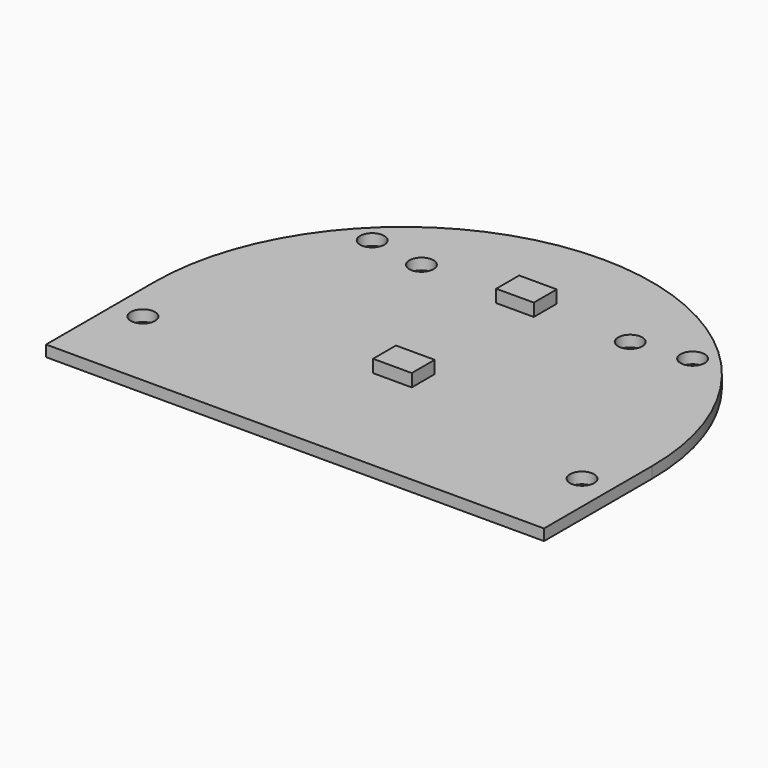
from build123d import *

# Parameters (mm, degrees)
F0_W     = 66.9
F0_H     = 51.6
F1_DEPTH = 1.5
F2_R     = 33.44999
F3_R     = 1.625
F4_DEPTH = 1.5
F5_W     = 5.2
F5_H     = 3.85
F5_W_2   = 5.05
F6_DEPTH = 1.7


# Not quite as in the source:
# - a fillet or chamfer is up to 0.001 mm smaller than in the source, because OpenCascade refuses the exact size


with BuildPart() as f1:
    # F0 (on Top) → F1 (new body)
    with BuildSketch(Plane.XY):
        Rectangle(F0_W, F0_H)
    extrude(amount=F1_DEPTH)

    # F2 (radius 33.45 in the source; OpenCascade refuses exactly that, so slightly less here)
    f2_edges = [f1.edges().sort_by_distance(p)[0] for p in [
        (-33.45, 25.8, 0.75),
        (33.45, 25.8, 0.75),
    ]]
    fillet(f2_edges, radius=F2_R)

    # F3 (on Top) → F4 (cut)
    with BuildSketch(Plane.XY):
        with Locations((-21.525, 14.0641658831)):
            Circle(F3_R)
        with Locations((-14.025, 12.9547324661)):
            Circle(F3_R)
        with Locations((21.525, 14.0641658831)):
            Circle(F3_R)
        with Locations((14.025, 12.9547324661)):
            Circle(F3_R)
        with Locations((-29.5, -14.475)):
            Circle(F3_R)
        with Locations((29.5, -14.475)):
            Circle(F3_R)
    extrude(amount=F4_DEPTH, mode=Mode.SUBTRACT)

    # F5 (on face) → F6 (join)
    with BuildSketch(Plane.XY.offset(1.5)):
        with Locations((0, -7.525)):
            Rectangle(F5_W, F5_H)
        with Locations((0.075, 12.975)):
            Rectangle(F5_W_2, F5_H)
    extrude(amount=F6_DEPTH)


solid = f1.part
